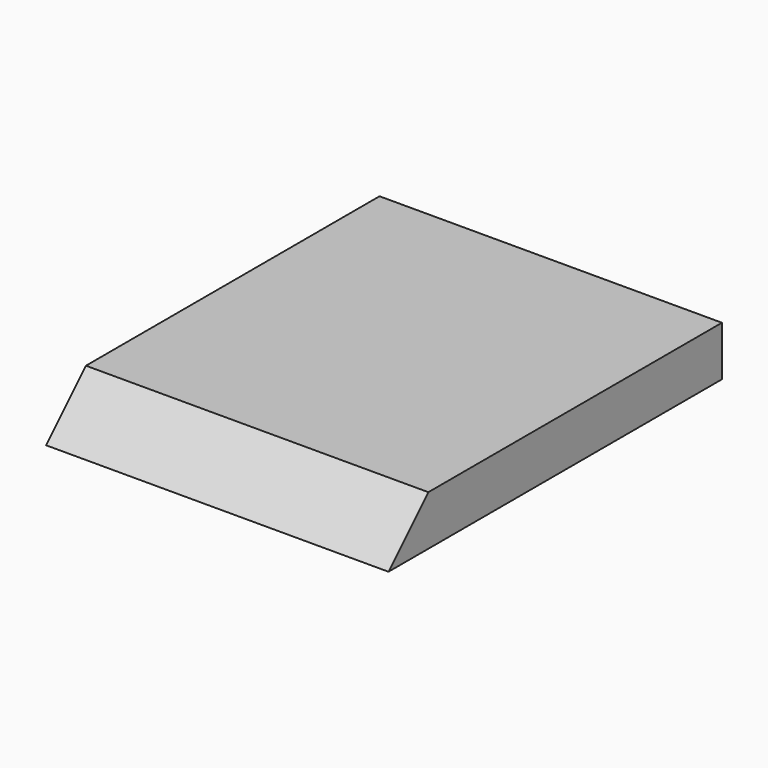
from build123d import *

# Parameters (mm, degrees)
F0_W     = 110
F0_H     = 133.888
F1_DEPTH = 16
F2_SIZE  = 15.99999


# Not quite as in the source:
# - a fillet or chamfer is up to 0.001 mm smaller than in the source, because OpenCascade refuses the exact size


with BuildPart() as f1:
    # F0 (on Top) → F1 (new body)
    with BuildSketch(Plane.XY):
        with Locations((55, 66.944)):
            Rectangle(F0_W, F0_H)
    extrude(amount=F1_DEPTH)

    # F2 (size 16 in the source; OpenCascade refuses exactly that, so slightly less here)
    f2_edges = [f1.edges().sort_by_distance(p)[0] for p in [
        (55, 0, 16),
    ]]
    chamfer(f2_edges, length=F2_SIZE)


solid = f1.part
